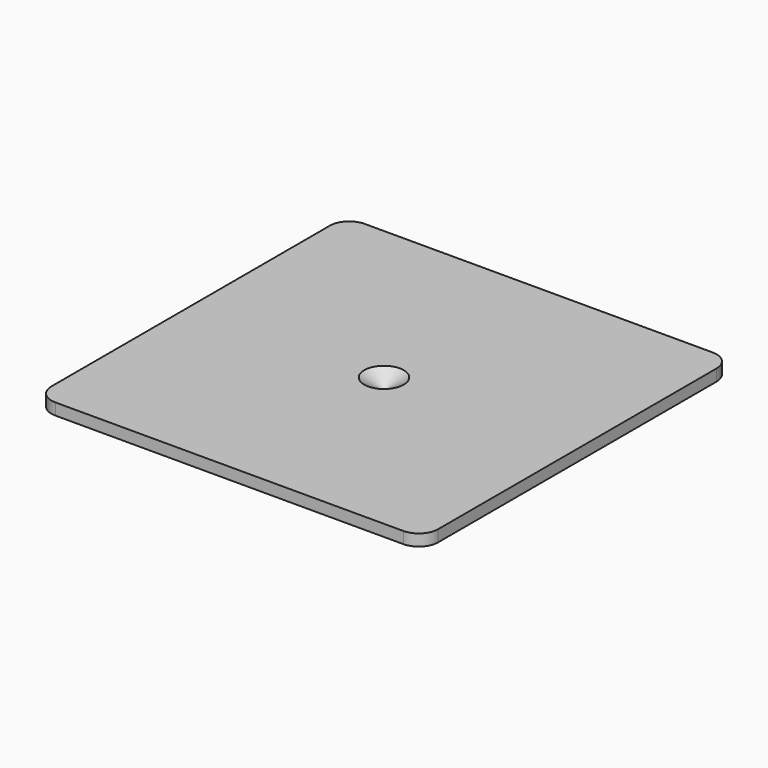
from build123d import *

# Parameters (mm, degrees)
F0_W     = 100
F0_H     = 100
F0_R     = 0.1
F1_DEPTH = 3
F2_SIZE2 = 2.99999
F2_SIZE  = 4.99999
F3_R     = 5


# Not quite as in the source:
# - a fillet or chamfer is up to 0.001 mm smaller than in the source, because OpenCascade refuses the exact size


with BuildPart() as f1:
    # F0 (on Top) → F1 (new body)
    with BuildSketch(Plane.XY):
        Rectangle(F0_W, F0_H)
        Circle(F0_R, mode=Mode.SUBTRACT)
    extrude(amount=F1_DEPTH)

    # F2 (size 5 and 3 in the source; OpenCascade refuses exactly that, so slightly less here)
    f2_edges = [f1.edges().sort_by_distance(p)[0] for p in [
        (-0.1, 0, 3),
    ]]
    f2_side = f1.faces().sort_by_distance((0, -48.585786, 3))[0]
    chamfer(f2_edges, length=F2_SIZE, length2=F2_SIZE2, reference=f2_side)

    # F3
    f3_edges = [f1.edges().sort_by_distance(p)[0] for p in [
        (50, -50, 1.5),
        (-50, -50, 1.5),
        (50, 50, 1.5),
        (-50, 50, 1.5),
    ]]
    fillet(f3_edges, radius=F3_R)


solid = f1.part
